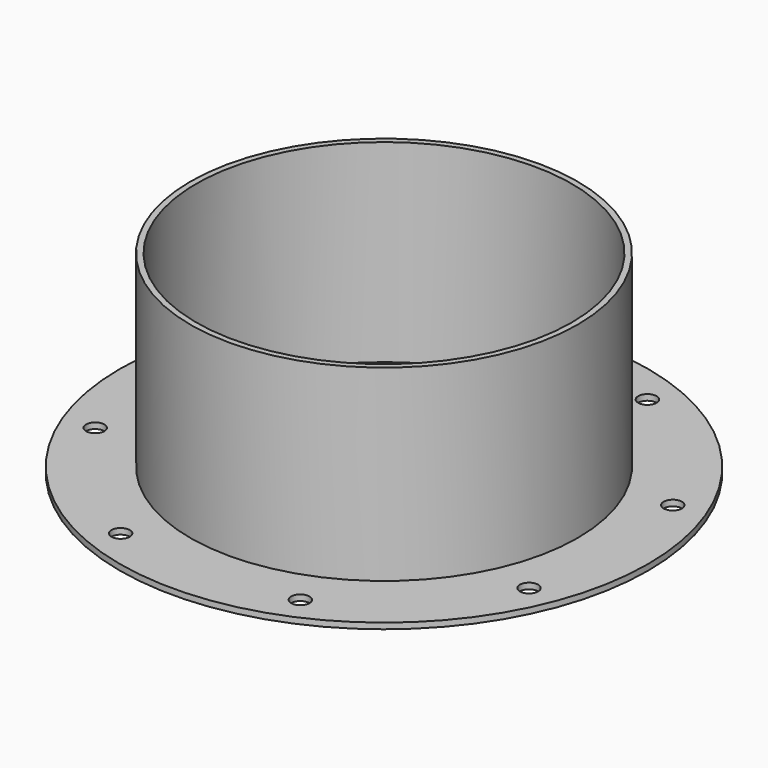
from build123d import *

# Parameters (mm, degrees)
F0_R            = 104.775
F0_R_2          = 101.6
F1_DEPTH        = 101.6
F2_R            = 142.875
F2_R_2          = 101.6
F3_DEPTH        = 3.175
F5_D            = 9.921875
F5_COPIES_COUNT = 8


# Not quite as in the source:
# - a length typed as a fraction of an inch, garbled in the dataset ("3 / 203.2 mm" for 3/8 in), is restored
# - a pattern or mirror of a feature is missing from the dataset's text; its kind, count and spacing are read off the source's solid


with BuildPart() as f1:
    # F0 (on Top) → F1 (new body)
    with BuildSketch(Plane.XY):
        Circle(F0_R)
        Circle(F0_R_2, mode=Mode.SUBTRACT)
    extrude(amount=F1_DEPTH)

    # F2 (on face) → F3 (join)
    with BuildSketch(Plane(origin=(0, 0, 0), x_dir=(1, 0, 0), z_dir=(0, 0, -1))):
        Circle(F2_R)
        Circle(F2_R_2, mode=Mode.SUBTRACT)
    extrude(amount=F3_DEPTH)

    # F5 (through all)
    with Locations(Plane.XY):
        with Locations((117.3327006289, -48.6007959104)):
            f5 = Hole(F5_D / 2)

    # F5_copies: F5 ×8 about axis
    f5_copies_axis = Axis((0, 0, 0), (0, 0, 1))
    for i in range(1, F5_COPIES_COUNT):
        add(f5.rotate(f5_copies_axis, i * 360 / F5_COPIES_COUNT), mode=Mode.SUBTRACT)


solid = f1.part
